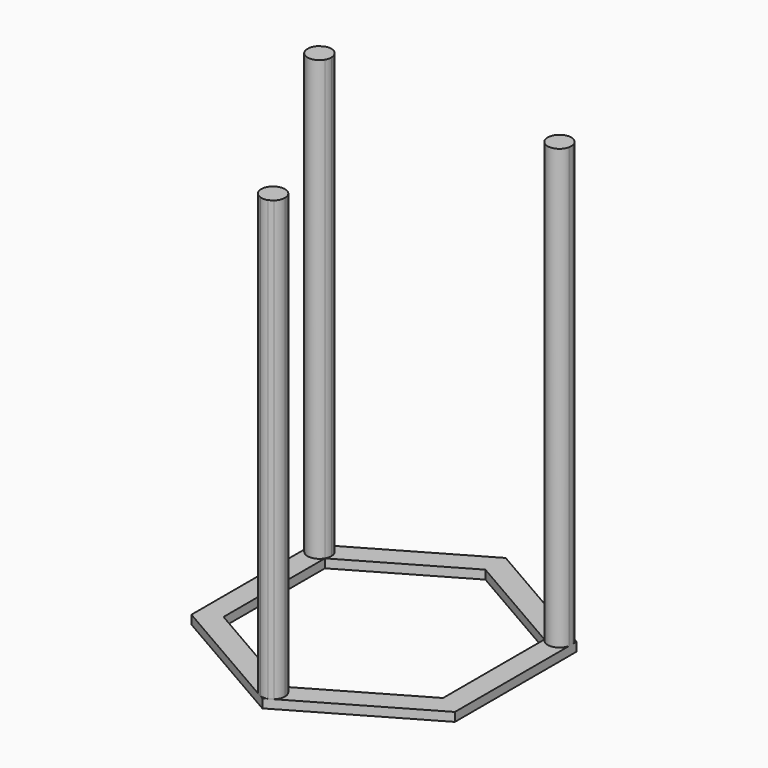
from build123d import *

# Parameters (mm, degrees)
F1_DEPTH = 2.54
F3_DEPTH = 127


# Not quite as in the source:
# - ends of sketch curves that miss each other by under 0.0002 mm in the source are joined


with BuildPart() as f1:
    # F0 (on Top) → F1 (new body)
    with BuildSketch(Plane.XY):
        Polygon((34.9249995572, 23.8301315939), (3.1749995572, 42.1610026407), (0, 43.994091056), (-38.1000004709, 21.997045528), (-38.1000004709, -21.997045528), (0, -43.994091056), (38.1000004709, -21.997045528), (38.1000004709, 21.997045528), align=None)
        Polygon((0, 36.6617420935), (31.75, 18.3308710468), (31.75, -18.3308710468), (0, -36.6617420935), (-31.75, -18.3308710468), (-31.75, 18.3308710468), align=None, mode=Mode.SUBTRACT)
    extrude(amount=F1_DEPTH)

    # F2 (on face) → F3 (join)
    with BuildSketch(Plane.XY.offset(2.54)):
        with BuildLine():
            ThreePointArc((-38.1000004709, 19.3844549358), (-35.2889631462, 16.6640411269), (-31.75, 18.3308710468))
            ThreePointArc((-31.75, 18.3308710468), (-31.403147802, 19.1639531761), (-31.2848175618, 20.0585649554))
            ThreePointArc((-31.2848175618, 20.0585649554), (-32.7035344951, 22.8425648101), (-35.7897937807, 23.3308439825))
            Line((-35.7897937807, 23.3308439825), (-37.0276020707, 22.616195033))
            ThreePointArc((-37.0276020707, 22.616195033), (-37.7159751418, 21.7610765108), (-38.1000004709, 20.7326749751))
            Line((-38.1000004709, 20.7326749751), (-38.1000004709, 19.3844549358))
        make_face()
        with BuildLine():
            ThreePointArc((35.8374259749, 23.3033424061), (32.0759629522, 22.2291160887), (31.75, 18.3308710468))
            ThreePointArc((31.75, 18.3308710468), (35.2686397989, 16.6449401257), (38.1000004709, 19.329448619))
            Line((38.1000004709, 19.329448619), (38.1000004709, 20.758746518))
            ThreePointArc((38.1000004709, 20.758746518), (37.7036332461, 21.7824533156), (37.0050252462, 22.6292292285))
            Line((37.0050252462, 22.6292292285), (35.8374259749, 23.3033424061))
        make_face()
        with BuildLine():
            ThreePointArc((3.4325778187, -40.1026625239), (2.4277039418, -37.6725121227), (0, -36.6617420935))
            ThreePointArc((0, -36.6617420935), (-3.2193789061, -38.8660080857), (-2.3102066902, -42.6602926015))
            Line((-2.3102066902, -42.6602926015), (-1.0723984002, -43.374941551))
            ThreePointArc((-1.0723984002, -43.374941551), (0.0123424988, -43.5435308567), (1.0949770186, -43.3619057795))
            Line((1.0949770186, -43.3619057795), (2.2625698225, -42.6877957599))
            ThreePointArc((2.2625698225, -42.6877957599), (3.1264590528, -41.5214500837), (3.4325778187, -40.1026625239))
        make_face()
    extrude(amount=F3_DEPTH)


solid = f1.part
